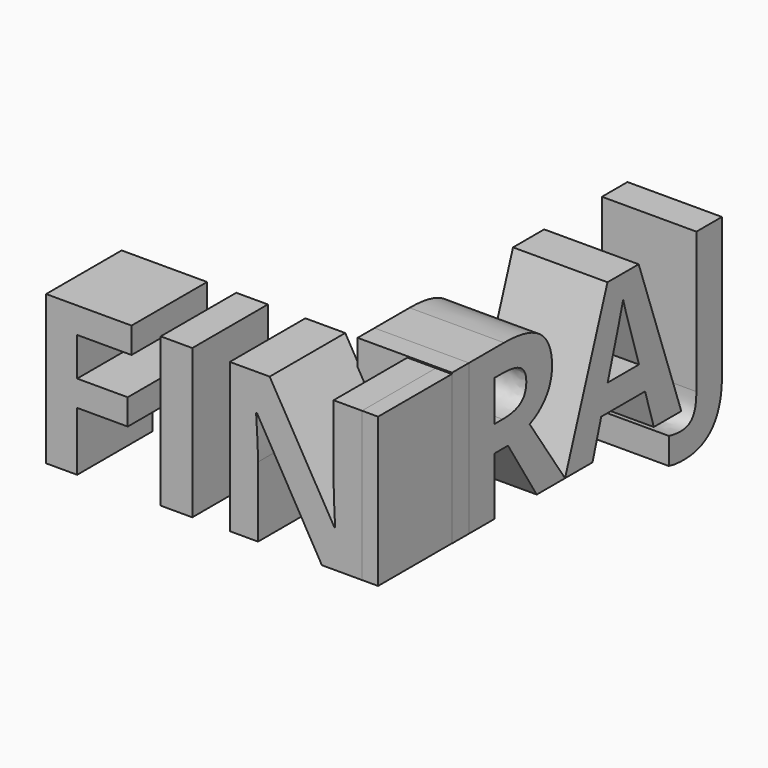
from build123d import *

# Parameters (mm, degrees)
F0_TEXT_SIZE = 28.0706367145
F2_DEPTH     = 12.7
F1_TEXT_SIZE = 28.3123692498
F3_DEPTH     = 12.7
F4_DEPTH     = 2.8448
F5_DEPTH     = 2.159


# Not quite as in the source:
# - Text() gives the source's letters only with a copy of the font that has no kerning and outlines rounded to 1/6400 em; it was checked with that copy


with BuildPart() as f2:
    # F0 (on Front) → F2 (new body)
    with BuildSketch(Plane.XZ):
        with Locations((-34.4834774733, 0)):
            Text('FIN', F0_TEXT_SIZE, font='Open Sans', font_style=FontStyle.BOLD, text_align=(TextAlign.LEFT, TextAlign.BOTTOM))
    extrude(amount=F2_DEPTH)


with BuildPart() as f3:
    # F1 (on Right) → F3 (new body)
    with BuildSketch(Plane.YZ):
        with Locations((0, 0)):
            Text('RAJ', F1_TEXT_SIZE, font='Open Sans', font_style=FontStyle.BOLD, text_align=(TextAlign.LEFT, TextAlign.BOTTOM))
    extrude(amount=F3_DEPTH)


with BuildPart() as f4:
    # F4 (new): a face of the model
    f4_faces = [f3.part.faces().sort_by_distance(p)[0] for p in [
        (6.35, 2.5436894248, 10.1061886799),
    ]]
    extrude(f4_faces, amount=F4_DEPTH)


with BuildPart() as f5:
    # F5 (new): a face of the model
    f5_faces = [f2.part.faces().sort_by_distance(p)[0] for p in [
        (10.5172620097, -6.35, 10.019901496),
    ]]
    extrude(f5_faces, amount=F5_DEPTH)


solid = Compound([f2.part, f3.part, f4.part, f5.part])
